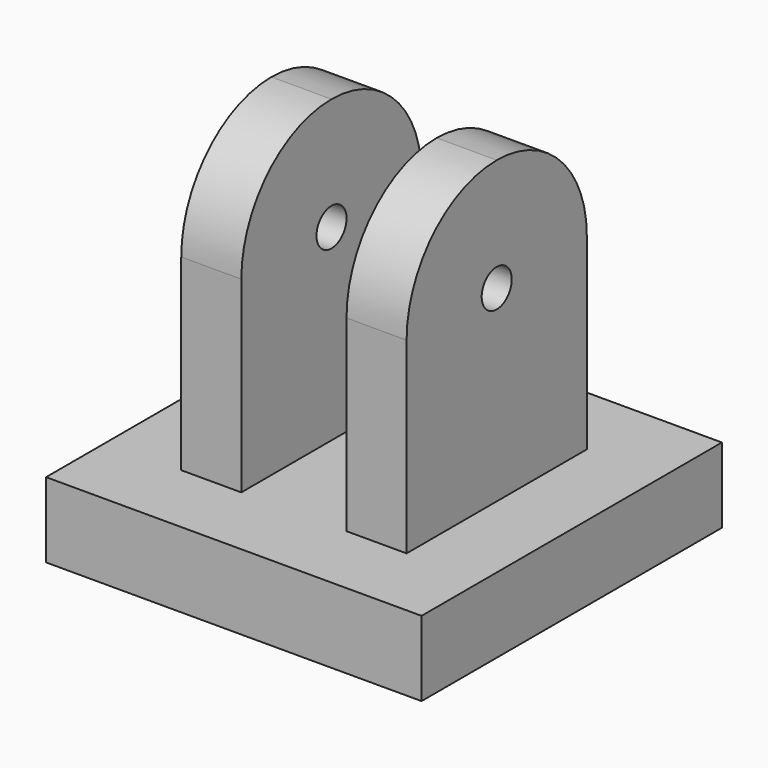
from build123d import *

# Parameters (mm, degrees)
F0_W     = 50
F0_H     = 50
F1_DEPTH = 10
F2_W     = 8
F2_H     = 30
F3_DEPTH = 40
F4_R     = 14.99999
F6_D     = 5


# Not quite as in the source:
# - a fillet or chamfer is up to 0.001 mm smaller than in the source, because OpenCascade refuses the exact size


with BuildPart() as f1:
    # F0 (on Top) → F1 (new body)
    with BuildSketch(Plane.XY):
        with Locations((1.9356412813, -0.2875153496)):
            Rectangle(F0_W, F0_H)
    extrude(amount=F1_DEPTH)

    # F2 (on face) → F3 (join)
    with BuildSketch(Plane.XY.offset(10)):
        with Locations((-9.0643587187, -0.2875153496)):
            Rectangle(F2_W, F2_H)
        with Locations((12.9356412813, -0.2770923451)):
            Rectangle(F2_W, F2_H)
    extrude(amount=F3_DEPTH)

    # F4 (radius 15 in the source; OpenCascade refuses exactly that, so slightly less here)
    f4_edges = [f1.edges().sort_by_distance(p)[0] for p in [
        (-9.064359, 14.712485, 50),
        (-9.064359, -15.287515, 50),
        (12.935641, 14.722908, 50),
        (12.935641, -15.277092, 50),
    ]]
    fillet(f4_edges, radius=F4_R)

    # F6 (through all)
    with Locations(Plane.YZ.offset(16.9356412813)):
        with Locations((-0.2770923451, 35)):
            Hole(F6_D / 2)


solid = f1.part
